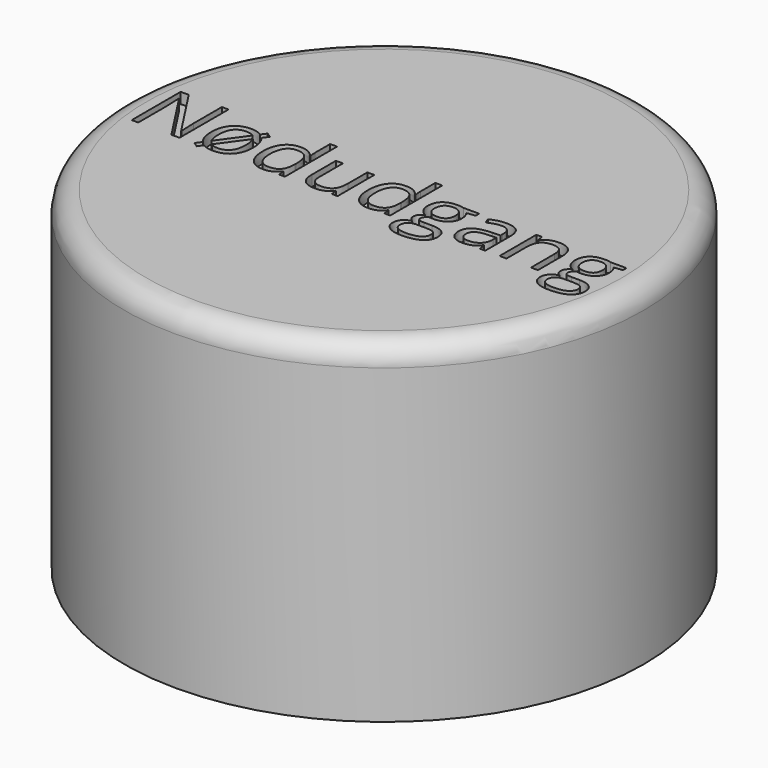
from build123d import *

# Parameters (mm, degrees)
F0_R         = 60
F1_DEPTH     = 77
F2_T         = -5
F3_R         = 5
F4_TEXT_SIZE = 19.8175153695
F5_DEPTH     = 2.5


# Not quite as in the source:
# - Text() gives the source's letters only with a copy of the font that has no kerning and outlines rounded to 1/6400 em; it was checked with that copy


with BuildPart() as f1:
    # F0 (on Top) → F1 (new body)
    with BuildSketch(Plane.XY):
        Circle(F0_R)
    extrude(amount=F1_DEPTH)

    # F2
    f2_openings = [f1.faces().sort_by_distance(p)[0] for p in [
        (0, 0, 0),
    ]]
    offset(amount=F2_T, openings=f2_openings)

    # F3
    f3_edges = [f1.edges().sort_by_distance(p)[0] for p in [
        (-60, 0, 77),
    ]]
    fillet(f3_edges, radius=F3_R)

    # F4 (on face) → F5 (cut)
    with BuildSketch(Plane.XY.offset(77)):
        with Locations((-54.5353251073, -7.134305533)):
            Text('Nødudgang', F4_TEXT_SIZE, font='Open Sans', text_align=(TextAlign.LEFT, TextAlign.BOTTOM))
    extrude(amount=-F5_DEPTH, mode=Mode.SUBTRACT)


solid = f1.part
